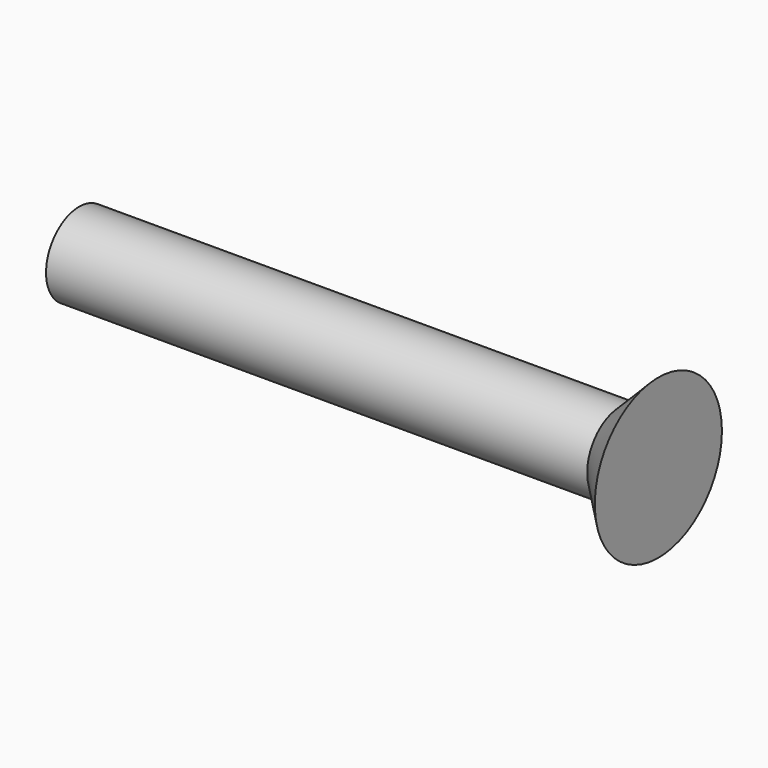
from build123d import *

# Parameters (mm, degrees)
F0_R        = 2.5
F1_DEPTH    = 35
F2_R        = 5
F2_R_2      = 2.5
F3_DEPTH    = 2.8
F4_S5_R     = 2.5
F4_T6_DEPTH = 9


# Not quite as in the source:
# - a fillet or chamfer that OpenCascade refuses, or shapes differently, is made with other operations: its cross-section is extruded or revolved along the edge and cut away or added


with BuildPart() as f1:
    # F0 (on Right) → F1 (new body)
    with BuildSketch(Plane.YZ):
        Circle(F0_R)
    extrude(amount=F1_DEPTH)

    # F2 (on face) → F3 (join)
    with BuildSketch(Plane.YZ.offset(35)):
        Circle(F2_R)
        Circle(F2_R_2, mode=Mode.SUBTRACT)
    extrude(amount=-F3_DEPTH)

    # F4: chamfer of 3 on 1 edges, made by hand


with BuildPart() as f4_tool2:
    # F4_s3 → F4_t4 (revolve)
    with BuildSketch(Plane.XY):
        Polygon((32.2, 2), (35.2, 5), (32.2, 5), align=None)
    revolve(axis=Axis((32.2, 0, 0), (1, 0, 0)))

    # F4_s5 → F4_t6 (cut, symmetric)
    with BuildSketch(Plane.YZ.offset(33.7)):
        Circle(F4_S5_R)
    extrude(amount=F4_T6_DEPTH, both=True, mode=Mode.SUBTRACT)


with BuildPart() as f1_1:
    add(f1.part)

    # F4_t1: cut F4_tool2
    add(f4_tool2.part, mode=Mode.SUBTRACT)


solid = f1_1.part
